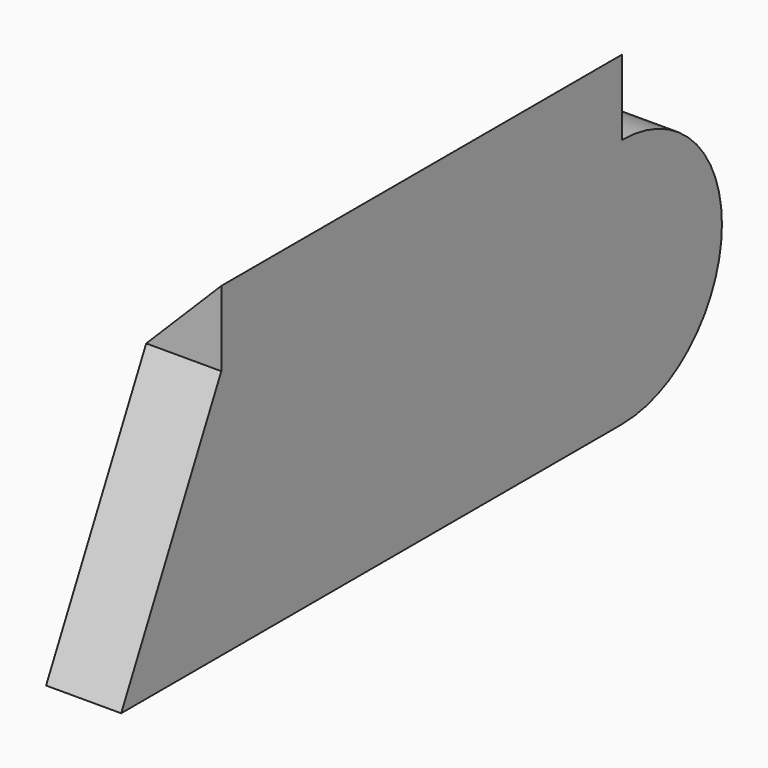
from build123d import *

# Parameters (mm, degrees)
F1_DEPTH = 15.24
F2_DEPTH = 12.7
F3_DEPTH = 15.24
F5_DEPTH = 228.6


# Not quite as in the source:
# - a feature names something its author has since deleted; it is built from what else it names


with BuildPart() as f1:
    # F0 (on Right) → F1 (new body)
    with BuildSketch(Plane.YZ):
        with BuildLine():
            ThreePointArc((37.1756509936, -4.7328671039), (19.2151387515, 2.7066206539), (11.7756509936, 20.6671328961))
            Line((11.7756509936, 20.6671328961), (-77.1243490064, 20.6671328961))
            Line((-77.1243490064, 20.6671328961), (-89.8243490064, -4.7328671039))
            Line((-89.8243490064, -4.7328671039), (37.1756509936, -4.7328671039))
        make_face()
        with BuildLine():
            Line((-77.1243490064, 20.6671328961), (11.7756509936, 20.6671328961))
            ThreePointArc((11.7756509936, 20.6671328961), (19.2151387515, 38.6276451382), (37.1756509936, 46.0671328961))
            Line((37.1756509936, 46.0671328961), (-64.4243490064, 46.0671328961))
            Line((-64.4243490064, 46.0671328961), (-77.1243490064, 20.6671328961))
        make_face()
    extrude(amount=-F1_DEPTH)

    # F0 (on Right) → F2 (join)
    with BuildSketch(Plane.YZ):
        with BuildLine():
            Line((11.7756509936, 20.6671328961), (62.5756509936, 20.6671328961))
            ThreePointArc((62.5756509936, 20.6671328961), (55.1361632357, 38.6276451382), (37.1756509936, 46.0671328961))
            ThreePointArc((37.1756509936, 46.0671328961), (19.2151387515, 38.6276451382), (11.7756509936, 20.6671328961))
        make_face()
        with BuildLine():
            ThreePointArc((37.1756509936, -4.7328671039), (55.1361632357, 2.7066206539), (62.5756509936, 20.6671328961))
            Line((62.5756509936, 20.6671328961), (11.7756509936, 20.6671328961))
            ThreePointArc((11.7756509936, 20.6671328961), (19.2151387515, 2.7066206539), (37.1756509936, -4.7328671039))
        make_face()
    extrude(amount=-F2_DEPTH)

    # F3 (add): a face of the model
    f3_faces = [f1.faces().sort_by_distance(p)[0] for p in [
        (-7.62, -13.6243490064, 46.0671328961),
    ]]
    extrude(f3_faces, amount=F3_DEPTH)

    # F4 (on face) → F5 (cut)
    with BuildSketch(Plane.XZ.offset(64.4243490064)):
        Polygon((-15.24, 46.0671328961), (0, 61.3071328961), (-15.24, 61.3071328961), align=None)
    extrude(amount=-F5_DEPTH, mode=Mode.SUBTRACT)


solid = f1.part
